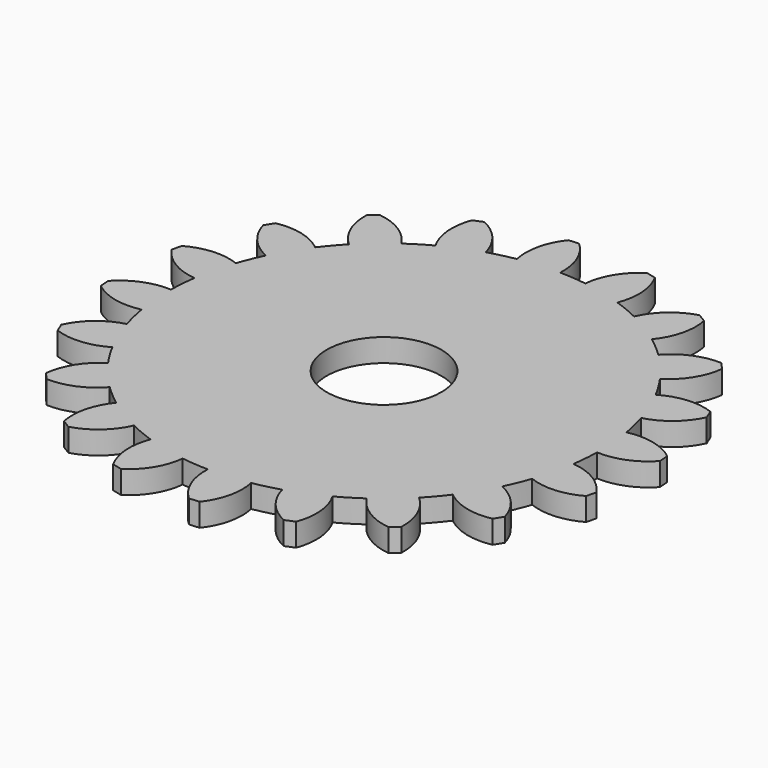
from build123d import *

# Parameters (mm, degrees)
F2_R     = 2.5
F3_DEPTH = 1


# Not quite as in the source:
# - a feature of the source that left no trace in its solid (it failed there, or was rolled back) is left out


with BuildPart() as f3:
    # F2 (on Top) → F3 (new body)
    with BuildSketch(Plane.XY):
        with BuildLine():
            ThreePointArc((-1.6229776334, 9.2680599554), (-0.7382287643, 9.3800858219), (0.1531520845, 9.4078443957))
            ThreePointArc((0.1531520845, 9.4078443957), (-0.0317997207, 10.5374998224), (-0.6817601701, 11.4797736507))
            Line((-0.6817601701, 11.4797736507), (-1.1224656787, 11.4450893749))
            ThreePointArc((-1.1224656787, 11.4450893749), (-1.6170199342, 10.4127402859), (-1.6229776334, 9.2680599554))
        make_face()
        with BuildLine():
            ThreePointArc((9.4078443957, -0.1531520845), (9.4087792756, -0.0765785786), (9.4090909091, 0))
            ThreePointArc((9.4090909091, 0), (9.3737668631, 0.8145468262), (9.2680599554, 1.6229776334))
            ThreePointArc((9.2680599554, 1.6229776334), (9.1491169783, 2.1965086508), (8.9947183137, 2.7615275108))
            ThreePointArc((8.9947183137, 2.7615275108), (8.6928665104, 3.6007032045), (8.3129211438, 4.4075314852))
            ThreePointArc((8.3129211438, 4.4075314852), (8.0225688191, 4.9162364953), (7.7011265332, 5.4058895526))
            ThreePointArc((7.7011265332, 5.4058895526), (7.1547288581, 6.1107157275), (6.5440556911, 6.7606454461))
            ThreePointArc((6.5440556911, 6.7606454461), (6.1107157275, 7.1547288581), (5.6536948308, 7.52108546))
            ThreePointArc((5.6536948308, 7.52108546), (4.9162364953, 8.0225688191), (4.1346124722, 8.4519803265))
            ThreePointArc((4.1346124722, 8.4519803265), (3.6007032045, 8.6928665104), (3.0528400867, 8.90006512))
            ThreePointArc((3.0528400867, 8.90006512), (2.1965086508, 9.1491169783), (1.320444577, 9.3159764842))
            ThreePointArc((1.320444577, 9.3159764842), (0.7382287643, 9.3800858219), (0.1531520845, 9.4078443957))
            ThreePointArc((0.1531520845, 9.4078443957), (-0.7382287643, 9.3800858219), (-1.6229776334, 9.2680599554))
            ThreePointArc((-1.6229776334, 9.2680599554), (-2.1965086508, 9.1491169783), (-2.7615275108, 8.9947183137))
            ThreePointArc((-2.7615275108, 8.9947183137), (-3.6007032045, 8.6928665104), (-4.4075314852, 8.3129211438))
            ThreePointArc((-4.4075314852, 8.3129211438), (-4.9162364953, 8.0225688191), (-5.4058895526, 7.7011265332))
            ThreePointArc((-5.4058895526, 7.7011265332), (-6.1107157275, 7.1547288581), (-6.7606454461, 6.5440556911))
            ThreePointArc((-6.7606454461, 6.5440556911), (-7.1547288581, 6.1107157275), (-7.52108546, 5.6536948308))
            ThreePointArc((-7.52108546, 5.6536948308), (-8.0225688191, 4.9162364953), (-8.4519803265, 4.1346124722))
            ThreePointArc((-8.4519803265, 4.1346124722), (-8.6928665104, 3.6007032045), (-8.90006512, 3.0528400867))
            ThreePointArc((-8.90006512, 3.0528400867), (-9.1491169783, 2.1965086508), (-9.3159764842, 1.320444577))
            ThreePointArc((-9.3159764842, 1.320444577), (-9.3800858219, 0.7382287643), (-9.4078443957, 0.1531520845))
            ThreePointArc((-9.4078443957, 0.1531520845), (-9.3800858219, -0.7382287643), (-9.2680599554, -1.6229776334))
            ThreePointArc((-9.2680599554, -1.6229776334), (-9.1491169783, -2.1965086508), (-8.9947183137, -2.7615275108))
            ThreePointArc((-8.9947183137, -2.7615275108), (-8.6928665104, -3.6007032045), (-8.3129211438, -4.4075314852))
            ThreePointArc((-8.3129211438, -4.4075314852), (-8.0225688191, -4.9162364953), (-7.7011265332, -5.4058895526))
            ThreePointArc((-7.7011265332, -5.4058895526), (-7.1547288581, -6.1107157275), (-6.5440556911, -6.7606454461))
            ThreePointArc((-6.5440556911, -6.7606454461), (-6.1107157275, -7.1547288581), (-5.6536948308, -7.52108546))
            ThreePointArc((-5.6536948308, -7.52108546), (-4.9162364953, -8.0225688191), (-4.1346124722, -8.4519803265))
            ThreePointArc((-4.1346124722, -8.4519803265), (-3.6007032045, -8.6928665104), (-3.0528400867, -8.90006512))
            ThreePointArc((-3.0528400867, -8.90006512), (-2.1965086508, -9.1491169783), (-1.320444577, -9.3159764842))
            ThreePointArc((-1.320444577, -9.3159764842), (-0.7382287643, -9.3800858219), (-0.1531520845, -9.4078443957))
            ThreePointArc((-0.1531520845, -9.4078443957), (0.7382287643, -9.3800858219), (1.6229776334, -9.2680599554))
            ThreePointArc((1.6229776334, -9.2680599554), (2.1965086508, -9.1491169783), (2.7615275108, -8.9947183137))
            ThreePointArc((2.7615275108, -8.9947183137), (3.6007032045, -8.6928665104), (4.4075314852, -8.3129211438))
            ThreePointArc((4.4075314852, -8.3129211438), (4.9162364953, -8.0225688191), (5.4058895526, -7.7011265332))
            ThreePointArc((5.4058895526, -7.7011265332), (6.1107157275, -7.1547288581), (6.7606454461, -6.5440556911))
            ThreePointArc((6.7606454461, -6.5440556911), (7.1547288581, -6.1107157275), (7.52108546, -5.6536948308))
            ThreePointArc((7.52108546, -5.6536948308), (8.0225688191, -4.9162364953), (8.4519803265, -4.1346124722))
            ThreePointArc((8.4519803265, -4.1346124722), (8.6928665104, -3.6007032045), (8.90006512, -3.0528400867))
            ThreePointArc((8.90006512, -3.0528400867), (9.1491169783, -2.1965086508), (9.3159764842, -1.320444577))
            ThreePointArc((9.3159764842, -1.320444577), (9.3800858219, -0.7382287643), (9.4078443957, -0.1531520845))
        make_face()
        Circle(F2_R, mode=Mode.SUBTRACT)
        with BuildLine():
            ThreePointArc((-4.4075314852, 8.3129211438), (-3.6007032045, 8.6928665104), (-2.7615275108, 8.9947183137))
            ThreePointArc((-2.7615275108, 8.9947183137), (-3.286509855, 10.0119312174), (-4.195837602, 10.7072380574))
            Line((-4.195837602, 10.7072380574), (-4.604255417, 10.5380658593))
            ThreePointArc((-4.604255417, 10.5380658593), (-4.7555910517, 9.4034178615), (-4.4075314852, 8.3129211438))
        make_face()
        with BuildLine():
            ThreePointArc((-6.7606454461, 6.5440556911), (-6.1107157275, 7.1547288581), (-5.4058895526, 7.7011265332))
            ThreePointArc((-5.4058895526, 7.7011265332), (-6.2195135061, 8.5063250277), (-7.2991972152, 8.8866034014))
            Line((-7.2991972152, 8.8866034014), (-7.6353485554, 8.5995030343))
            ThreePointArc((-7.6353485554, 8.5995030343), (-7.428651783, 7.4736233793), (-6.7606454461, 6.5440556911))
        make_face()
        with BuildLine():
            ThreePointArc((-8.4519803265, 4.1346124722), (-8.0225688191, 4.9162364953), (-7.52108546, 5.6536948308))
            ThreePointArc((-7.52108546, 5.6536948308), (-8.5437078414, 6.1680604771), (-9.6880605486, 6.1960860878))
            Line((-9.6880605486, 6.1960860878), (-9.9190405786, 5.8191609361))
            ThreePointArc((-9.9190405786, 5.8191609361), (-9.3745443193, 4.812258569), (-8.4519803265, 4.1346124722))
        make_face()
        with BuildLine():
            ThreePointArc((-9.3159764842, 1.320444577), (-9.1491169783, 2.1965086508), (-8.90006512, 3.0528400867))
            ThreePointArc((-8.90006512, 3.0528400867), (-10.0315845257, 3.2260231917), (-11.1285890147, 2.8990526973))
            Line((-11.1285890147, 2.8990526973), (-11.2317877999, 2.469198821))
            ThreePointArc((-11.2317877999, 2.469198821), (-10.4027911413, 1.679836361), (-9.3159764842, 1.320444577))
        make_face()
        with BuildLine():
            ThreePointArc((-9.2680599554, -1.6229776334), (-9.3800858219, -0.7382287643), (-9.4078443957, 0.1531520845))
            ThreePointArc((-9.4078443957, 0.1531520845), (-10.5374998224, -0.0317997207), (-11.4797736507, -0.6817601701))
            Line((-11.4797736507, -0.6817601701), (-11.4450893749, -1.1224656787))
            ThreePointArc((-11.4450893749, -1.1224656787), (-10.4127402859, -1.6170199342), (-9.2680599554, -1.6229776334))
        make_face()
        with BuildLine():
            ThreePointArc((-10.5380658593, -4.604255417), (-9.4034178615, -4.7555910517), (-8.3129211438, -4.4075314852))
            ThreePointArc((-8.3129211438, -4.4075314852), (-8.6928665104, -3.6007032045), (-8.9947183137, -2.7615275108))
            ThreePointArc((-8.9947183137, -2.7615275108), (-10.0119312174, -3.286509855), (-10.7072380574, -4.195837602))
            Line((-10.7072380574, -4.195837602), (-10.5380658593, -4.604255417))
        make_face()
        with BuildLine():
            ThreePointArc((-8.5995030343, -7.6353485554), (-7.4736233793, -7.428651783), (-6.5440556911, -6.7606454461))
            ThreePointArc((-6.5440556911, -6.7606454461), (-7.1547288581, -6.1107157275), (-7.7011265332, -5.4058895526))
            ThreePointArc((-7.7011265332, -5.4058895526), (-8.5063250277, -6.2195135061), (-8.8866034014, -7.2991972152))
            Line((-8.8866034014, -7.2991972152), (-8.5995030343, -7.6353485554))
        make_face()
        with BuildLine():
            ThreePointArc((-5.8191609361, -9.9190405786), (-4.812258569, -9.3745443193), (-4.1346124722, -8.4519803265))
            ThreePointArc((-4.1346124722, -8.4519803265), (-4.9162364953, -8.0225688191), (-5.6536948308, -7.52108546))
            ThreePointArc((-5.6536948308, -7.52108546), (-6.1680604771, -8.5437078414), (-6.1960860878, -9.6880605486))
            Line((-6.1960860878, -9.6880605486), (-5.8191609361, -9.9190405786))
        make_face()
        with BuildLine():
            ThreePointArc((-2.469198821, -11.2317877999), (-1.679836361, -10.4027911413), (-1.320444577, -9.3159764842))
            ThreePointArc((-1.320444577, -9.3159764842), (-2.1965086508, -9.1491169783), (-3.0528400867, -8.90006512))
            ThreePointArc((-3.0528400867, -8.90006512), (-3.2260231917, -10.0315845257), (-2.8990526973, -11.1285890147))
            Line((-2.8990526973, -11.1285890147), (-2.469198821, -11.2317877999))
        make_face()
        with BuildLine():
            ThreePointArc((1.1224656787, -11.4450893749), (1.6170199342, -10.4127402859), (1.6229776334, -9.2680599554))
            ThreePointArc((1.6229776334, -9.2680599554), (0.7382287643, -9.3800858219), (-0.1531520845, -9.4078443957))
            ThreePointArc((-0.1531520845, -9.4078443957), (0.0317997207, -10.5374998224), (0.6817601701, -11.4797736507))
            Line((0.6817601701, -11.4797736507), (1.1224656787, -11.4450893749))
        make_face()
        with BuildLine():
            ThreePointArc((4.604255417, -10.5380658593), (4.7555910517, -9.4034178615), (4.4075314852, -8.3129211438))
            ThreePointArc((4.4075314852, -8.3129211438), (3.6007032045, -8.6928665104), (2.7615275108, -8.9947183137))
            ThreePointArc((2.7615275108, -8.9947183137), (3.286509855, -10.0119312174), (4.195837602, -10.7072380574))
            Line((4.195837602, -10.7072380574), (4.604255417, -10.5380658593))
        make_face()
        with BuildLine():
            ThreePointArc((7.6353485554, -8.5995030343), (7.428651783, -7.4736233793), (6.7606454461, -6.5440556911))
            ThreePointArc((6.7606454461, -6.5440556911), (6.1107157275, -7.1547288581), (5.4058895526, -7.7011265332))
            ThreePointArc((5.4058895526, -7.7011265332), (6.2195135061, -8.5063250277), (7.2991972152, -8.8866034014))
            Line((7.2991972152, -8.8866034014), (7.6353485554, -8.5995030343))
        make_face()
        with BuildLine():
            ThreePointArc((9.9190405786, -5.8191609361), (9.3745443193, -4.812258569), (8.4519803265, -4.1346124722))
            ThreePointArc((8.4519803265, -4.1346124722), (8.0225688191, -4.9162364953), (7.52108546, -5.6536948308))
            ThreePointArc((7.52108546, -5.6536948308), (8.5437078414, -6.1680604771), (9.6880605486, -6.1960860878))
            Line((9.6880605486, -6.1960860878), (9.9190405786, -5.8191609361))
        make_face()
        with BuildLine():
            ThreePointArc((11.2317877999, -2.469198821), (10.4027911413, -1.679836361), (9.3159764842, -1.320444577))
            ThreePointArc((9.3159764842, -1.320444577), (9.1491169783, -2.1965086508), (8.90006512, -3.0528400867))
            ThreePointArc((8.90006512, -3.0528400867), (10.0315845257, -3.2260231917), (11.1285890147, -2.8990526973))
            Line((11.1285890147, -2.8990526973), (11.2317877999, -2.469198821))
        make_face()
        with BuildLine():
            ThreePointArc((9.2680599554, 1.6229776334), (9.3737668631, 0.8145468262), (9.4090909091, 0))
            ThreePointArc((9.4090909091, 0), (9.4087792756, -0.0765785786), (9.4078443957, -0.1531520845))
            ThreePointArc((9.4078443957, -0.1531520845), (10.5374998224, 0.0317997207), (11.4797736507, 0.6817601701))
            Line((11.4797736507, 0.6817601701), (11.4450893749, 1.1224656787))
            ThreePointArc((11.4450893749, 1.1224656787), (10.4127402859, 1.6170199342), (9.2680599554, 1.6229776334))
        make_face()
        with BuildLine():
            ThreePointArc((8.3129211438, 4.4075314852), (8.6928665104, 3.6007032045), (8.9947183137, 2.7615275108))
            ThreePointArc((8.9947183137, 2.7615275108), (10.0119312174, 3.286509855), (10.7072380574, 4.195837602))
            Line((10.7072380574, 4.195837602), (10.5380658593, 4.604255417))
            ThreePointArc((10.5380658593, 4.604255417), (9.4034178615, 4.7555910517), (8.3129211438, 4.4075314852))
        make_face()
        with BuildLine():
            ThreePointArc((6.5440556911, 6.7606454461), (7.1547288581, 6.1107157275), (7.7011265332, 5.4058895526))
            ThreePointArc((7.7011265332, 5.4058895526), (8.5063250277, 6.2195135061), (8.8866034014, 7.2991972152))
            Line((8.8866034014, 7.2991972152), (8.5995030343, 7.6353485554))
            ThreePointArc((8.5995030343, 7.6353485554), (7.4736233793, 7.428651783), (6.5440556911, 6.7606454461))
        make_face()
        with BuildLine():
            ThreePointArc((4.1346124722, 8.4519803265), (4.9162364953, 8.0225688191), (5.6536948308, 7.52108546))
            ThreePointArc((5.6536948308, 7.52108546), (6.1680604771, 8.5437078414), (6.1960860878, 9.6880605486))
            Line((6.1960860878, 9.6880605486), (5.8191609361, 9.9190405786))
            ThreePointArc((5.8191609361, 9.9190405786), (4.812258569, 9.3745443193), (4.1346124722, 8.4519803265))
        make_face()
        with BuildLine():
            ThreePointArc((1.320444577, 9.3159764842), (2.1965086508, 9.1491169783), (3.0528400867, 8.90006512))
            ThreePointArc((3.0528400867, 8.90006512), (3.2260231917, 10.0315845257), (2.8990526973, 11.1285890147))
            Line((2.8990526973, 11.1285890147), (2.469198821, 11.2317877999))
            ThreePointArc((2.469198821, 11.2317877999), (1.679836361, 10.4027911413), (1.320444577, 9.3159764842))
        make_face()
    extrude(amount=F3_DEPTH)


solid = f3.part
